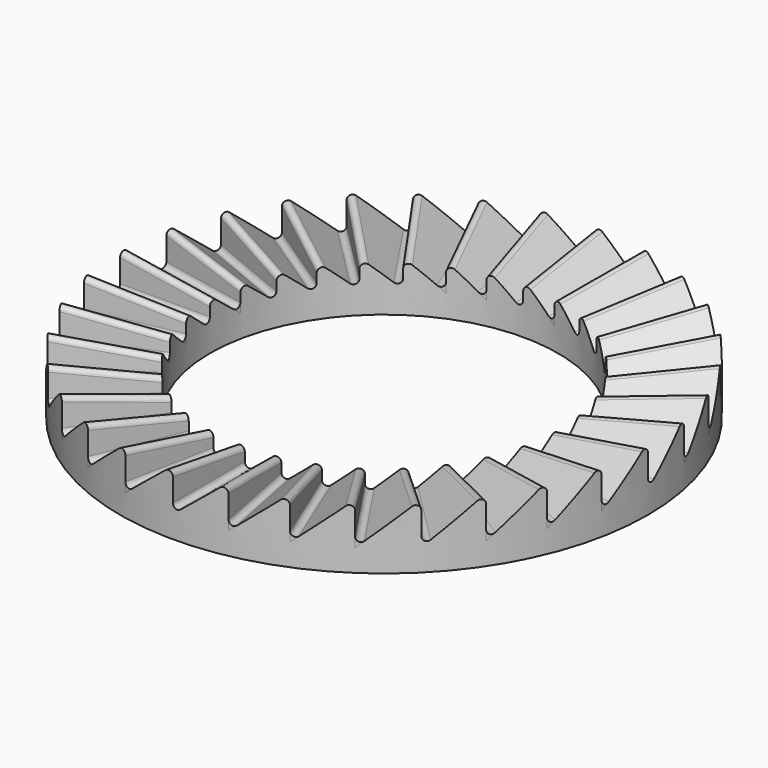
from build123d import *

# Parameters (mm, degrees)
F0_R          = 23.5
F0_R_2        = 15.5
F1_DEPTH      = 10
F3_DEPTH      = 23.5
F4_COUNT      = 32
F4_ANGLE      = 348.75
F7_T4_DEPTH   = 12.2119902172
F7_S5_R       = 23.5
F7_T6_DEPTH   = 8
F7_S7_R       = 15.5
F7_T8_DEPTH   = 8
F7_T12_DEPTH  = 12.2119902172
F7_S13_R      = 23.5
F7_T14_DEPTH  = 8
F7_S15_R      = 15.5
F7_T16_DEPTH  = 8
F7_T20_DEPTH  = 12.2119902172
F7_S21_R      = 23.5
F7_T22_DEPTH  = 8
F7_S23_R      = 15.5
F7_T24_DEPTH  = 8
F7_T28_DEPTH  = 12.2119902172
F7_S29_R      = 23.5
F7_T30_DEPTH  = 8
F7_S31_R      = 15.5
F7_T32_DEPTH  = 8
F7_T36_DEPTH  = 12.2119902172
F7_S37_R      = 23.5
F7_T38_DEPTH  = 8
F7_S39_R      = 15.5
F7_T40_DEPTH  = 8
F7_T44_DEPTH  = 12.2119902172
F7_S45_R      = 23.5
F7_T46_DEPTH  = 8
F7_S47_R      = 15.5
F7_T48_DEPTH  = 8
F7_T52_DEPTH  = 12.2119902172
F7_S53_R      = 23.5
F7_T54_DEPTH  = 8
F7_S55_R      = 15.5
F7_T56_DEPTH  = 8
F7_T60_DEPTH  = 12.2119902172
F7_S61_R      = 23.5
F7_T62_DEPTH  = 8
F7_S63_R      = 15.5
F7_T64_DEPTH  = 8
F7_T68_DEPTH  = 12.2119902172
F7_S69_R      = 23.5
F7_T70_DEPTH  = 8
F7_S71_R      = 15.5
F7_T72_DEPTH  = 8
F7_T76_DEPTH  = 12.2119902172
F7_S77_R      = 23.5
F7_T78_DEPTH  = 8
F7_S79_R      = 15.5
F7_T80_DEPTH  = 8
F7_T84_DEPTH  = 12.2119902172
F7_S85_R      = 23.5
F7_T86_DEPTH  = 8
F7_S87_R      = 15.5
F7_T88_DEPTH  = 8
F7_T92_DEPTH  = 12.2119902172
F7_S93_R      = 23.5
F7_T94_DEPTH  = 8
F7_S95_R      = 15.5
F7_T96_DEPTH  = 8
F7_T100_DEPTH = 12.2119902172
F7_S101_R     = 23.5
F7_T102_DEPTH = 8
F7_S103_R     = 15.5
F7_T104_DEPTH = 8
F7_T108_DEPTH = 12.2119902172
F7_S109_R     = 23.5
F7_T110_DEPTH = 8
F7_S111_R     = 15.5
F7_T112_DEPTH = 8
F7_T116_DEPTH = 12.2119902172
F7_S117_R     = 23.5
F7_T118_DEPTH = 8
F7_S119_R     = 15.5
F7_T120_DEPTH = 8
F7_T124_DEPTH = 12.2119902172
F7_S125_R     = 23.5
F7_T126_DEPTH = 8
F7_S127_R     = 15.5
F7_T128_DEPTH = 8
F7_T132_DEPTH = 12.2119902172
F7_S133_R     = 23.5
F7_T134_DEPTH = 8
F7_S135_R     = 15.5
F7_T136_DEPTH = 8
F7_T140_DEPTH = 12.2119902172
F7_S141_R     = 23.5
F7_T142_DEPTH = 8
F7_S143_R     = 15.5
F7_T144_DEPTH = 8
F7_T148_DEPTH = 12.2119902172
F7_S149_R     = 23.5
F7_T150_DEPTH = 8
F7_S151_R     = 15.5
F7_T152_DEPTH = 8
F7_T156_DEPTH = 12.2119902172
F7_S157_R     = 23.5
F7_T158_DEPTH = 8
F7_S159_R     = 15.5
F7_T160_DEPTH = 8
F7_T164_DEPTH = 12.2119902172
F7_S165_R     = 23.5
F7_T166_DEPTH = 8
F7_S167_R     = 15.5
F7_T168_DEPTH = 8
F7_T172_DEPTH = 12.2119902172
F7_S173_R     = 23.5
F7_T174_DEPTH = 8
F7_S175_R     = 15.5
F7_T176_DEPTH = 8
F7_T180_DEPTH = 12.2119902172
F7_S181_R     = 23.5
F7_T182_DEPTH = 8
F7_S183_R     = 15.5
F7_T184_DEPTH = 8
F7_T188_DEPTH = 12.2119902172
F7_S189_R     = 23.5
F7_T190_DEPTH = 8
F7_S191_R     = 15.5
F7_T192_DEPTH = 8
F7_T196_DEPTH = 12.2119902172
F7_S197_R     = 23.5
F7_T198_DEPTH = 8
F7_S199_R     = 15.5
F7_T200_DEPTH = 8
F7_T204_DEPTH = 12.2119902172
F7_S205_R     = 23.5
F7_T206_DEPTH = 8
F7_S207_R     = 15.5
F7_T208_DEPTH = 8
F7_T212_DEPTH = 12.2119902172
F7_S213_R     = 23.5
F7_T214_DEPTH = 8
F7_S215_R     = 15.5
F7_T216_DEPTH = 8
F7_T220_DEPTH = 12.2119902172
F7_S221_R     = 23.5
F7_T222_DEPTH = 8
F7_S223_R     = 15.5
F7_T224_DEPTH = 8
F7_T228_DEPTH = 12.2119902172
F7_S229_R     = 23.5
F7_T230_DEPTH = 8
F7_S231_R     = 15.5
F7_T232_DEPTH = 8
F7_T236_DEPTH = 12.2119902172
F7_S237_R     = 23.5
F7_T238_DEPTH = 8
F7_S239_R     = 15.5
F7_T240_DEPTH = 8
F7_T244_DEPTH = 12.2119902172
F7_S245_R     = 23.5
F7_T246_DEPTH = 8
F7_S247_R     = 15.5
F7_T248_DEPTH = 8
F7_T252_DEPTH = 12.2119902172
F7_S253_R     = 23.5
F7_T254_DEPTH = 8
F7_S255_R     = 15.5
F7_T256_DEPTH = 8
F7_T257_DEPTH = 12.2293454889
F7_T259_DEPTH = 12.2293454889
F7_T261_DEPTH = 12.2293454889
F7_T263_DEPTH = 12.2293454889
F7_T265_DEPTH = 12.2293454889
F7_T267_DEPTH = 12.2293454889
F7_T269_DEPTH = 12.2293454889
F7_T271_DEPTH = 12.2293454889
F7_T273_DEPTH = 12.2293454889
F7_T275_DEPTH = 12.2293454889
F7_T277_DEPTH = 12.2293454889
F7_T279_DEPTH = 12.2293454889
F7_T281_DEPTH = 12.2293454889
F7_T283_DEPTH = 12.2293454889
F7_T285_DEPTH = 12.2293454889
F7_T287_DEPTH = 12.2293454889
F7_T289_DEPTH = 12.2293454889
F7_T291_DEPTH = 12.2293454889
F7_T293_DEPTH = 12.2293454889
F7_T295_DEPTH = 12.2293454889
F7_T297_DEPTH = 12.2293454889
F7_T299_DEPTH = 12.2293454889
F7_T301_DEPTH = 12.2293454889
F7_T303_DEPTH = 12.2293454889
F7_T305_DEPTH = 12.2293454889
F7_T307_DEPTH = 12.2293454889
F7_T309_DEPTH = 12.2293454889
F7_T311_DEPTH = 12.2293454889
F7_T313_DEPTH = 12.2293454889
F7_T315_DEPTH = 12.2293454889
F7_T317_DEPTH = 12.2293454889
F7_T319_DEPTH = 12.2293454889


# Not quite as in the source:
# - a fillet or chamfer that OpenCascade refuses, or shapes differently, is made with other operations: its cross-section is extruded or revolved along the edge and cut away or added


with BuildPart() as f1:
    # F0 (on Top) → F1 (new body)
    with BuildSketch(Plane.XY):
        Circle(F0_R)
        Circle(F0_R_2, mode=Mode.SUBTRACT)
    extrude(amount=F1_DEPTH)


with BuildPart() as f3:
    # F2 (on Right) → F3 (new body)
    with BuildSketch(Plane.YZ):
        Polygon((9.808969115, 10.0010584846), (0, 10.0010584846), (0, 2.0010584846), align=None)
    extrude(amount=F3_DEPTH)


with BuildPart() as f4_1:
    # F4: instance of F3
    add(f3.part.rotate(Axis((0, 0, 6.0010584846), (0, 0, -1)), 1 * F4_ANGLE / (F4_COUNT - 1)))


with BuildPart() as f4_2:
    # F4: instance of F3
    add(f3.part.rotate(Axis((0, 0, 6.0010584846), (0, 0, -1)), 2 * F4_ANGLE / (F4_COUNT - 1)))


with BuildPart() as f4_3:
    # F4: instance of F3
    add(f3.part.rotate(Axis((0, 0, 6.0010584846), (0, 0, -1)), 3 * F4_ANGLE / (F4_COUNT - 1)))


with BuildPart() as f4_4:
    # F4: instance of F3
    add(f3.part.rotate(Axis((0, 0, 6.0010584846), (0, 0, -1)), 4 * F4_ANGLE / (F4_COUNT - 1)))


with BuildPart() as f4_5:
    # F4: instance of F3
    add(f3.part.rotate(Axis((0, 0, 6.0010584846), (0, 0, -1)), 5 * F4_ANGLE / (F4_COUNT - 1)))


with BuildPart() as f4_6:
    # F4: instance of F3
    add(f3.part.rotate(Axis((0, 0, 6.0010584846), (0, 0, -1)), 6 * F4_ANGLE / (F4_COUNT - 1)))


with BuildPart() as f4_7:
    # F4: instance of F3
    add(f3.part.rotate(Axis((0, 0, 6.0010584846), (0, 0, -1)), 7 * F4_ANGLE / (F4_COUNT - 1)))


with BuildPart() as f4_8:
    # F4: instance of F3
    add(f3.part.rotate(Axis((0, 0, 6.0010584846), (0, 0, -1)), 8 * F4_ANGLE / (F4_COUNT - 1)))


with BuildPart() as f4_9:
    # F4: instance of F3
    add(f3.part.rotate(Axis((0, 0, 6.0010584846), (0, 0, -1)), 9 * F4_ANGLE / (F4_COUNT - 1)))


with BuildPart() as f4_10:
    # F4: instance of F3
    add(f3.part.rotate(Axis((0, 0, 6.0010584846), (0, 0, -1)), 10 * F4_ANGLE / (F4_COUNT - 1)))


with BuildPart() as f4_11:
    # F4: instance of F3
    add(f3.part.rotate(Axis((0, 0, 6.0010584846), (0, 0, -1)), 11 * F4_ANGLE / (F4_COUNT - 1)))


with BuildPart() as f4_12:
    # F4: instance of F3
    add(f3.part.rotate(Axis((0, 0, 6.0010584846), (0, 0, -1)), 12 * F4_ANGLE / (F4_COUNT - 1)))


with BuildPart() as f4_13:
    # F4: instance of F3
    add(f3.part.rotate(Axis((0, 0, 6.0010584846), (0, 0, -1)), 13 * F4_ANGLE / (F4_COUNT - 1)))


with BuildPart() as f4_14:
    # F4: instance of F3
    add(f3.part.rotate(Axis((0, 0, 6.0010584846), (0, 0, -1)), 14 * F4_ANGLE / (F4_COUNT - 1)))


with BuildPart() as f4_15:
    # F4: instance of F3
    add(f3.part.rotate(Axis((0, 0, 6.0010584846), (0, 0, -1)), 15 * F4_ANGLE / (F4_COUNT - 1)))


with BuildPart() as f4_16:
    # F4: instance of F3
    add(f3.part.rotate(Axis((0, 0, 6.0010584846), (0, 0, -1)), 16 * F4_ANGLE / (F4_COUNT - 1)))


with BuildPart() as f4_17:
    # F4: instance of F3
    add(f3.part.rotate(Axis((0, 0, 6.0010584846), (0, 0, -1)), 17 * F4_ANGLE / (F4_COUNT - 1)))


with BuildPart() as f4_18:
    # F4: instance of F3
    add(f3.part.rotate(Axis((0, 0, 6.0010584846), (0, 0, -1)), 18 * F4_ANGLE / (F4_COUNT - 1)))


with BuildPart() as f4_19:
    # F4: instance of F3
    add(f3.part.rotate(Axis((0, 0, 6.0010584846), (0, 0, -1)), 19 * F4_ANGLE / (F4_COUNT - 1)))


with BuildPart() as f4_20:
    # F4: instance of F3
    add(f3.part.rotate(Axis((0, 0, 6.0010584846), (0, 0, -1)), 20 * F4_ANGLE / (F4_COUNT - 1)))


with BuildPart() as f4_21:
    # F4: instance of F3
    add(f3.part.rotate(Axis((0, 0, 6.0010584846), (0, 0, -1)), 21 * F4_ANGLE / (F4_COUNT - 1)))


with BuildPart() as f4_22:
    # F4: instance of F3
    add(f3.part.rotate(Axis((0, 0, 6.0010584846), (0, 0, -1)), 22 * F4_ANGLE / (F4_COUNT - 1)))


with BuildPart() as f4_23:
    # F4: instance of F3
    add(f3.part.rotate(Axis((0, 0, 6.0010584846), (0, 0, -1)), 23 * F4_ANGLE / (F4_COUNT - 1)))


with BuildPart() as f4_24:
    # F4: instance of F3
    add(f3.part.rotate(Axis((0, 0, 6.0010584846), (0, 0, -1)), 24 * F4_ANGLE / (F4_COUNT - 1)))


with BuildPart() as f4_25:
    # F4: instance of F3
    add(f3.part.rotate(Axis((0, 0, 6.0010584846), (0, 0, -1)), 25 * F4_ANGLE / (F4_COUNT - 1)))


with BuildPart() as f4_26:
    # F4: instance of F3
    add(f3.part.rotate(Axis((0, 0, 6.0010584846), (0, 0, -1)), 26 * F4_ANGLE / (F4_COUNT - 1)))


with BuildPart() as f4_27:
    # F4: instance of F3
    add(f3.part.rotate(Axis((0, 0, 6.0010584846), (0, 0, -1)), 27 * F4_ANGLE / (F4_COUNT - 1)))


with BuildPart() as f4_28:
    # F4: instance of F3
    add(f3.part.rotate(Axis((0, 0, 6.0010584846), (0, 0, -1)), 28 * F4_ANGLE / (F4_COUNT - 1)))


with BuildPart() as f4_29:
    # F4: instance of F3
    add(f3.part.rotate(Axis((0, 0, 6.0010584846), (0, 0, -1)), 29 * F4_ANGLE / (F4_COUNT - 1)))


with BuildPart() as f4_30:
    # F4: instance of F3
    add(f3.part.rotate(Axis((0, 0, 6.0010584846), (0, 0, -1)), 30 * F4_ANGLE / (F4_COUNT - 1)))


with BuildPart() as f4_31:
    # F4: instance of F3
    add(f3.part.rotate(Axis((0, 0, 6.0010584846), (0, 0, -1)), 31 * F4_ANGLE / (F4_COUNT - 1)))


with BuildPart() as f3_1:
    add(f3.part)

    # F5: union F4_1, F4_2, F4_3, F4_4, F4_5, F4_6, F4_7, F4_8, F4_9, F4_10, F4_11, F4_12, F4_13, F4_14, F4_15, F4_16, F4_17, F4_18, F4_19, F4_20, F4_21, F4_22, F4_23, F4_24, F4_25, F4_26, F4_27, F4_28, F4_29, F4_30, F4_31
    add(f4_1.part)
    add(f4_2.part)
    add(f4_3.part)
    add(f4_4.part)
    add(f4_5.part)
    add(f4_6.part)
    add(f4_7.part)
    add(f4_8.part)
    add(f4_9.part)
    add(f4_10.part)
    add(f4_11.part)
    add(f4_12.part)
    add(f4_13.part)
    add(f4_14.part)
    add(f4_15.part)
    add(f4_16.part)
    add(f4_17.part)
    add(f4_18.part)
    add(f4_19.part)
    add(f4_20.part)
    add(f4_21.part)
    add(f4_22.part)
    add(f4_23.part)
    add(f4_24.part)
    add(f4_25.part)
    add(f4_26.part)
    add(f4_27.part)
    add(f4_28.part)
    add(f4_29.part)
    add(f4_30.part)
    add(f4_31.part)


with BuildPart() as f1_1:
    add(f1.part)

    # F6: cut F3
    add(f3_1.part, mode=Mode.SUBTRACT)

    # F7: fillet of radius 0.4 on 64 edges, made by hand


with BuildPart() as f7_tool2:
    # F7_s3 → F7_t4 (new body)
    with BuildSketch(Plane(origin=(5.1256637649, -12.3744469775, 0), x_dir=(0, 0, 1), z_dir=(0.3826834324, -0.9238795325, 0))):
        with BuildLine():
            add(Edge.make_bspline(
                [(2.5334787325, -0.6528117211), (2.0010584846, 0), (2.843456528, 0)],
                knots=[0, 0, 0, 1, 1, 1], degree=2, weights=[1, 0.4285714286, 1]))
            Line((2.843456528, 0), (2.0010584846, 0))
            Line((2.0010584846, 0), (2.5334787325, -0.6528117211))
        make_face()
    extrude(amount=F7_T4_DEPTH)

    # F7_s5 → F7_t6 (intersect, symmetric)
    with BuildSketch(Plane.XY.offset(2.4)):
        Circle(F7_S5_R)
    extrude(amount=F7_T6_DEPTH, both=True, mode=Mode.INTERSECT)

    # F7_s7 → F7_t8 (cut, symmetric)
    with BuildSketch(Plane.XY.offset(2.4)):
        Circle(F7_S7_R)
    extrude(amount=F7_T8_DEPTH, both=True, mode=Mode.SUBTRACT)


with BuildPart() as f1_2:
    add(f1_1.part)

    # F7_t1: union F7_tool2
    add(f7_tool2.part)


with BuildPart() as f7_tool10:
    # F7_s11 → F7_t12 (new body)
    with BuildSketch(Plane(origin=(7.4413104186, -11.1367080542, 0), x_dir=(0, 0, 1), z_dir=(0.555570233, -0.8314696123, 0))):
        with BuildLine():
            add(Edge.make_bspline(
                [(2.5334787325, -0.6528117211), (2.0010584846, 0), (2.843456528, 0)],
                knots=[0, 0, 0, 1, 1, 1], degree=2, weights=[1, 0.4285714286, 1]))
            Line((2.843456528, 0), (2.0010584846, 0))
            Line((2.0010584846, 0), (2.5334787325, -0.6528117211))
        make_face()
    extrude(amount=F7_T12_DEPTH)

    # F7_s13 → F7_t14 (intersect, symmetric)
    with BuildSketch(Plane.XY.offset(2.4)):
        Circle(F7_S13_R)
    extrude(amount=F7_T14_DEPTH, both=True, mode=Mode.INTERSECT)

    # F7_s15 → F7_t16 (cut, symmetric)
    with BuildSketch(Plane.XY.offset(2.4)):
        Circle(F7_S15_R)
    extrude(amount=F7_T16_DEPTH, both=True, mode=Mode.SUBTRACT)


with BuildPart() as f1_3:
    add(f1_2.part)

    # F7_t9: union F7_tool10
    add(f7_tool10.part)


with BuildPart() as f7_tool18:
    # F7_s19 → F7_t20 (new body)
    with BuildSketch(Plane(origin=(9.4709916859, -9.4709916859, 0), x_dir=(0, 0, 1), z_dir=(0.7071067812, -0.7071067812, 0))):
        with BuildLine():
            add(Edge.make_bspline(
                [(2.5334787325, -0.6528117211), (2.0010584846, 0), (2.843456528, 0)],
                knots=[0, 0, 0, 1, 1, 1], degree=2, weights=[1, 0.4285714286, 1]))
            Line((2.843456528, 0), (2.0010584846, 0))
            Line((2.0010584846, 0), (2.5334787325, -0.6528117211))
        make_face()
    extrude(amount=F7_T20_DEPTH)

    # F7_s21 → F7_t22 (intersect, symmetric)
    with BuildSketch(Plane.XY.offset(2.4)):
        Circle(F7_S21_R)
    extrude(amount=F7_T22_DEPTH, both=True, mode=Mode.INTERSECT)

    # F7_s23 → F7_t24 (cut, symmetric)
    with BuildSketch(Plane.XY.offset(2.4)):
        Circle(F7_S23_R)
    extrude(amount=F7_T24_DEPTH, both=True, mode=Mode.SUBTRACT)


with BuildPart() as f1_4:
    add(f1_3.part)

    # F7_t17: union F7_tool18
    add(f7_tool18.part)


with BuildPart() as f7_tool26:
    # F7_s27 → F7_t28 (new body)
    with BuildSketch(Plane(origin=(11.1367080542, -7.4413104186, 0), x_dir=(0, 0, 1), z_dir=(0.8314696123, -0.555570233, 0))):
        with BuildLine():
            add(Edge.make_bspline(
                [(2.5334787325, -0.6528117211), (2.0010584846, 0), (2.843456528, 0)],
                knots=[0, 0, 0, 1, 1, 1], degree=2, weights=[1, 0.4285714286, 1]))
            Line((2.843456528, 0), (2.0010584846, 0))
            Line((2.0010584846, 0), (2.5334787325, -0.6528117211))
        make_face()
    extrude(amount=F7_T28_DEPTH)

    # F7_s29 → F7_t30 (intersect, symmetric)
    with BuildSketch(Plane.XY.offset(2.4)):
        Circle(F7_S29_R)
    extrude(amount=F7_T30_DEPTH, both=True, mode=Mode.INTERSECT)

    # F7_s31 → F7_t32 (cut, symmetric)
    with BuildSketch(Plane.XY.offset(2.4)):
        Circle(F7_S31_R)
    extrude(amount=F7_T32_DEPTH, both=True, mode=Mode.SUBTRACT)


with BuildPart() as f1_5:
    add(f1_4.part)

    # F7_t25: union F7_tool26
    add(f7_tool26.part)


with BuildPart() as f7_tool34:
    # F7_s35 → F7_t36 (new body)
    with BuildSketch(Plane(origin=(12.3744469775, -5.1256637649, 0), x_dir=(0, 0, 1), z_dir=(0.9238795325, -0.3826834324, 0))):
        with BuildLine():
            add(Edge.make_bspline(
                [(2.5334787325, -0.6528117211), (2.0010584846, 0), (2.843456528, 0)],
                knots=[0, 0, 0, 1, 1, 1], degree=2, weights=[1, 0.4285714286, 1]))
            Line((2.843456528, 0), (2.0010584846, 0))
            Line((2.0010584846, 0), (2.5334787325, -0.6528117211))
        make_face()
    extrude(amount=F7_T36_DEPTH)

    # F7_s37 → F7_t38 (intersect, symmetric)
    with BuildSketch(Plane.XY.offset(2.4)):
        Circle(F7_S37_R)
    extrude(amount=F7_T38_DEPTH, both=True, mode=Mode.INTERSECT)

    # F7_s39 → F7_t40 (cut, symmetric)
    with BuildSketch(Plane.XY.offset(2.4)):
        Circle(F7_S39_R)
    extrude(amount=F7_T40_DEPTH, both=True, mode=Mode.SUBTRACT)


with BuildPart() as f1_6:
    add(f1_5.part)

    # F7_t33: union F7_tool34
    add(f7_tool34.part)


with BuildPart() as f7_tool42:
    # F7_s43 → F7_t44 (new body)
    with BuildSketch(Plane(origin=(13.1366428431, -2.6130407273, 0), x_dir=(0, 0, 1), z_dir=(0.9807852804, -0.195090322, 0))):
        with BuildLine():
            add(Edge.make_bspline(
                [(2.5334787325, -0.6528117211), (2.0010584846, 0), (2.843456528, 0)],
                knots=[0, 0, 0, 1, 1, 1], degree=2, weights=[1, 0.4285714286, 1]))
            Line((2.843456528, 0), (2.0010584846, 0))
            Line((2.0010584846, 0), (2.5334787325, -0.6528117211))
        make_face()
    extrude(amount=F7_T44_DEPTH)

    # F7_s45 → F7_t46 (intersect, symmetric)
    with BuildSketch(Plane.XY.offset(2.4)):
        Circle(F7_S45_R)
    extrude(amount=F7_T46_DEPTH, both=True, mode=Mode.INTERSECT)

    # F7_s47 → F7_t48 (cut, symmetric)
    with BuildSketch(Plane.XY.offset(2.4)):
        Circle(F7_S47_R)
    extrude(amount=F7_T48_DEPTH, both=True, mode=Mode.SUBTRACT)


with BuildPart() as f1_7:
    add(f1_6.part)

    # F7_t41: union F7_tool42
    add(f7_tool42.part)


with BuildPart() as f7_tool50:
    # F7_s51 → F7_t52 (new body)
    with BuildSketch(Plane.YZ.offset(13.3940048914)):
        with BuildLine():
            add(Edge.make_bspline(
                [(0, 2.843456528), (0, 2.0010584846), (0.6528117211, 2.5334787325)],
                knots=[0, 0, 0, 1, 1, 1], degree=2, weights=[1, 0.4285714286, 1]))
            Line((0.6528117211, 2.5334787325), (0, 2.0010584846))
            Line((0, 2.0010584846), (0, 2.843456528))
        make_face()
    extrude(amount=F7_T52_DEPTH)

    # F7_s53 → F7_t54 (intersect, symmetric)
    with BuildSketch(Plane.XY.offset(2.4)):
        Circle(F7_S53_R)
    extrude(amount=F7_T54_DEPTH, both=True, mode=Mode.INTERSECT)

    # F7_s55 → F7_t56 (cut, symmetric)
    with BuildSketch(Plane.XY.offset(2.4)):
        Circle(F7_S55_R)
    extrude(amount=F7_T56_DEPTH, both=True, mode=Mode.SUBTRACT)


with BuildPart() as f1_8:
    add(f1_7.part)

    # F7_t49: union F7_tool50
    add(f7_tool50.part)


with BuildPart() as f7_tool58:
    # F7_s59 → F7_t60 (new body)
    with BuildSketch(Plane(origin=(13.1366428431, 2.6130407273, 0), x_dir=(0, 0, 1), z_dir=(0.9807852804, 0.195090322, 0))):
        with BuildLine():
            add(Edge.make_bspline(
                [(2.5334787325, -0.6528117211), (2.0010584846, 0), (2.843456528, 0)],
                knots=[0, 0, 0, 1, 1, 1], degree=2, weights=[1, 0.4285714286, 1]))
            Line((2.843456528, 0), (2.0010584846, 0))
            Line((2.0010584846, 0), (2.5334787325, -0.6528117211))
        make_face()
    extrude(amount=F7_T60_DEPTH)

    # F7_s61 → F7_t62 (intersect, symmetric)
    with BuildSketch(Plane.XY.offset(2.4)):
        Circle(F7_S61_R)
    extrude(amount=F7_T62_DEPTH, both=True, mode=Mode.INTERSECT)

    # F7_s63 → F7_t64 (cut, symmetric)
    with BuildSketch(Plane.XY.offset(2.4)):
        Circle(F7_S63_R)
    extrude(amount=F7_T64_DEPTH, both=True, mode=Mode.SUBTRACT)


with BuildPart() as f1_9:
    add(f1_8.part)

    # F7_t57: union F7_tool58
    add(f7_tool58.part)


with BuildPart() as f7_tool66:
    # F7_s67 → F7_t68 (new body)
    with BuildSketch(Plane(origin=(11.1367080542, 7.4413104186, 0), x_dir=(0, 0, 1), z_dir=(0.8314696123, 0.555570233, 0))):
        with BuildLine():
            add(Edge.make_bspline(
                [(2.5334787325, -0.6528117211), (2.0010584846, 0), (2.843456528, 0)],
                knots=[0, 0, 0, 1, 1, 1], degree=2, weights=[1, 0.4285714286, 1]))
            Line((2.843456528, 0), (2.0010584846, 0))
            Line((2.0010584846, 0), (2.5334787325, -0.6528117211))
        make_face()
    extrude(amount=F7_T68_DEPTH)

    # F7_s69 → F7_t70 (intersect, symmetric)
    with BuildSketch(Plane.XY.offset(2.4)):
        Circle(F7_S69_R)
    extrude(amount=F7_T70_DEPTH, both=True, mode=Mode.INTERSECT)

    # F7_s71 → F7_t72 (cut, symmetric)
    with BuildSketch(Plane.XY.offset(2.4)):
        Circle(F7_S71_R)
    extrude(amount=F7_T72_DEPTH, both=True, mode=Mode.SUBTRACT)


with BuildPart() as f1_10:
    add(f1_9.part)

    # F7_t65: union F7_tool66
    add(f7_tool66.part)


with BuildPart() as f7_tool74:
    # F7_s75 → F7_t76 (new body)
    with BuildSketch(Plane(origin=(12.3744469775, 5.1256637649, 0), x_dir=(0, 0, 1), z_dir=(0.9238795325, 0.3826834324, 0))):
        with BuildLine():
            add(Edge.make_bspline(
                [(2.5334787325, -0.6528117211), (2.0010584846, 0), (2.843456528, 0)],
                knots=[0, 0, 0, 1, 1, 1], degree=2, weights=[1, 0.4285714286, 1]))
            Line((2.843456528, 0), (2.0010584846, 0))
            Line((2.0010584846, 0), (2.5334787325, -0.6528117211))
        make_face()
    extrude(amount=F7_T76_DEPTH)

    # F7_s77 → F7_t78 (intersect, symmetric)
    with BuildSketch(Plane.XY.offset(2.4)):
        Circle(F7_S77_R)
    extrude(amount=F7_T78_DEPTH, both=True, mode=Mode.INTERSECT)

    # F7_s79 → F7_t80 (cut, symmetric)
    with BuildSketch(Plane.XY.offset(2.4)):
        Circle(F7_S79_R)
    extrude(amount=F7_T80_DEPTH, both=True, mode=Mode.SUBTRACT)


with BuildPart() as f1_11:
    add(f1_10.part)

    # F7_t73: union F7_tool74
    add(f7_tool74.part)


with BuildPart() as f7_tool82:
    # F7_s83 → F7_t84 (new body)
    with BuildSketch(Plane(origin=(9.4709916859, 9.4709916859, 0), x_dir=(0, 0, 1), z_dir=(0.7071067812, 0.7071067812, 0))):
        with BuildLine():
            add(Edge.make_bspline(
                [(2.5334787325, -0.6528117211), (2.0010584846, 0), (2.843456528, 0)],
                knots=[0, 0, 0, 1, 1, 1], degree=2, weights=[1, 0.4285714286, 1]))
            Line((2.843456528, 0), (2.0010584846, 0))
            Line((2.0010584846, 0), (2.5334787325, -0.6528117211))
        make_face()
    extrude(amount=F7_T84_DEPTH)

    # F7_s85 → F7_t86 (intersect, symmetric)
    with BuildSketch(Plane.XY.offset(2.4)):
        Circle(F7_S85_R)
    extrude(amount=F7_T86_DEPTH, both=True, mode=Mode.INTERSECT)

    # F7_s87 → F7_t88 (cut, symmetric)
    with BuildSketch(Plane.XY.offset(2.4)):
        Circle(F7_S87_R)
    extrude(amount=F7_T88_DEPTH, both=True, mode=Mode.SUBTRACT)


with BuildPart() as f1_12:
    add(f1_11.part)

    # F7_t81: union F7_tool82
    add(f7_tool82.part)


with BuildPart() as f7_tool90:
    # F7_s91 → F7_t92 (new body)
    with BuildSketch(Plane(origin=(7.4413104186, 11.1367080542, 0), x_dir=(0, 0, 1), z_dir=(0.555570233, 0.8314696123, 0))):
        with BuildLine():
            add(Edge.make_bspline(
                [(2.5334787325, -0.6528117211), (2.0010584846, 0), (2.843456528, 0)],
                knots=[0, 0, 0, 1, 1, 1], degree=2, weights=[1, 0.4285714286, 1]))
            Line((2.843456528, 0), (2.0010584846, 0))
            Line((2.0010584846, 0), (2.5334787325, -0.6528117211))
        make_face()
    extrude(amount=F7_T92_DEPTH)

    # F7_s93 → F7_t94 (intersect, symmetric)
    with BuildSketch(Plane.XY.offset(2.4)):
        Circle(F7_S93_R)
    extrude(amount=F7_T94_DEPTH, both=True, mode=Mode.INTERSECT)

    # F7_s95 → F7_t96 (cut, symmetric)
    with BuildSketch(Plane.XY.offset(2.4)):
        Circle(F7_S95_R)
    extrude(amount=F7_T96_DEPTH, both=True, mode=Mode.SUBTRACT)


with BuildPart() as f1_13:
    add(f1_12.part)

    # F7_t89: union F7_tool90
    add(f7_tool90.part)


with BuildPart() as f7_tool98:
    # F7_s99 → F7_t100 (new body)
    with BuildSketch(Plane(origin=(5.1256637649, 12.3744469775, 0), x_dir=(0, 0, 1), z_dir=(0.3826834324, 0.9238795325, 0))):
        with BuildLine():
            add(Edge.make_bspline(
                [(2.5334787325, -0.6528117211), (2.0010584846, 0), (2.843456528, 0)],
                knots=[0, 0, 0, 1, 1, 1], degree=2, weights=[1, 0.4285714286, 1]))
            Line((2.843456528, 0), (2.0010584846, 0))
            Line((2.0010584846, 0), (2.5334787325, -0.6528117211))
        make_face()
    extrude(amount=F7_T100_DEPTH)

    # F7_s101 → F7_t102 (intersect, symmetric)
    with BuildSketch(Plane.XY.offset(2.4)):
        Circle(F7_S101_R)
    extrude(amount=F7_T102_DEPTH, both=True, mode=Mode.INTERSECT)

    # F7_s103 → F7_t104 (cut, symmetric)
    with BuildSketch(Plane.XY.offset(2.4)):
        Circle(F7_S103_R)
    extrude(amount=F7_T104_DEPTH, both=True, mode=Mode.SUBTRACT)


with BuildPart() as f1_14:
    add(f1_13.part)

    # F7_t97: union F7_tool98
    add(f7_tool98.part)


with BuildPart() as f7_tool106:
    # F7_s107 → F7_t108 (new body)
    with BuildSketch(Plane(origin=(2.6130407273, 13.1366428431, 0), x_dir=(0, 0, 1), z_dir=(0.195090322, 0.9807852804, 0))):
        with BuildLine():
            add(Edge.make_bspline(
                [(2.5334787325, -0.6528117211), (2.0010584846, 0), (2.843456528, 0)],
                knots=[0, 0, 0, 1, 1, 1], degree=2, weights=[1, 0.4285714286, 1]))
            Line((2.843456528, 0), (2.0010584846, 0))
            Line((2.0010584846, 0), (2.5334787325, -0.6528117211))
        make_face()
    extrude(amount=F7_T108_DEPTH)

    # F7_s109 → F7_t110 (intersect, symmetric)
    with BuildSketch(Plane.XY.offset(2.4)):
        Circle(F7_S109_R)
    extrude(amount=F7_T110_DEPTH, both=True, mode=Mode.INTERSECT)

    # F7_s111 → F7_t112 (cut, symmetric)
    with BuildSketch(Plane.XY.offset(2.4)):
        Circle(F7_S111_R)
    extrude(amount=F7_T112_DEPTH, both=True, mode=Mode.SUBTRACT)


with BuildPart() as f1_15:
    add(f1_14.part)

    # F7_t105: union F7_tool106
    add(f7_tool106.part)


with BuildPart() as f7_tool114:
    # F7_s115 → F7_t116 (new body)
    with BuildSketch(Plane.XZ.offset(-13.3940048914)):
        with BuildLine():
            add(Edge.make_bspline(
                [(-0.6528117211, 2.5334787325), (0, 2.0010584846), (0, 2.843456528)],
                knots=[0, 0, 0, 1, 1, 1], degree=2, weights=[1, 0.4285714286, 1]))
            Line((0, 2.843456528), (0, 2.0010584846))
            Line((0, 2.0010584846), (-0.6528117211, 2.5334787325))
        make_face()
    extrude(amount=-F7_T116_DEPTH)

    # F7_s117 → F7_t118 (intersect, symmetric)
    with BuildSketch(Plane.XY.offset(2.4)):
        Circle(F7_S117_R)
    extrude(amount=F7_T118_DEPTH, both=True, mode=Mode.INTERSECT)

    # F7_s119 → F7_t120 (cut, symmetric)
    with BuildSketch(Plane.XY.offset(2.4)):
        Circle(F7_S119_R)
    extrude(amount=F7_T120_DEPTH, both=True, mode=Mode.SUBTRACT)


with BuildPart() as f1_16:
    add(f1_15.part)

    # F7_t113: union F7_tool114
    add(f7_tool114.part)


with BuildPart() as f7_tool122:
    # F7_s123 → F7_t124 (new body)
    with BuildSketch(Plane(origin=(-2.6130407273, 13.1366428431, 0), x_dir=(0, 0, 1), z_dir=(-0.195090322, 0.9807852804, 0))):
        with BuildLine():
            add(Edge.make_bspline(
                [(2.5334787325, -0.6528117211), (2.0010584846, 0), (2.843456528, 0)],
                knots=[0, 0, 0, 1, 1, 1], degree=2, weights=[1, 0.4285714286, 1]))
            Line((2.843456528, 0), (2.0010584846, 0))
            Line((2.0010584846, 0), (2.5334787325, -0.6528117211))
        make_face()
    extrude(amount=F7_T124_DEPTH)

    # F7_s125 → F7_t126 (intersect, symmetric)
    with BuildSketch(Plane.XY.offset(2.4)):
        Circle(F7_S125_R)
    extrude(amount=F7_T126_DEPTH, both=True, mode=Mode.INTERSECT)

    # F7_s127 → F7_t128 (cut, symmetric)
    with BuildSketch(Plane.XY.offset(2.4)):
        Circle(F7_S127_R)
    extrude(amount=F7_T128_DEPTH, both=True, mode=Mode.SUBTRACT)


with BuildPart() as f1_17:
    add(f1_16.part)

    # F7_t121: union F7_tool122
    add(f7_tool122.part)


with BuildPart() as f7_tool130:
    # F7_s131 → F7_t132 (new body)
    with BuildSketch(Plane(origin=(-5.1256637649, 12.3744469775, 0), x_dir=(0, 0, 1), z_dir=(-0.3826834324, 0.9238795325, 0))):
        with BuildLine():
            add(Edge.make_bspline(
                [(2.5334787325, -0.6528117211), (2.0010584846, 0), (2.843456528, 0)],
                knots=[0, 0, 0, 1, 1, 1], degree=2, weights=[1, 0.4285714286, 1]))
            Line((2.843456528, 0), (2.0010584846, 0))
            Line((2.0010584846, 0), (2.5334787325, -0.6528117211))
        make_face()
    extrude(amount=F7_T132_DEPTH)

    # F7_s133 → F7_t134 (intersect, symmetric)
    with BuildSketch(Plane.XY.offset(2.4)):
        Circle(F7_S133_R)
    extrude(amount=F7_T134_DEPTH, both=True, mode=Mode.INTERSECT)

    # F7_s135 → F7_t136 (cut, symmetric)
    with BuildSketch(Plane.XY.offset(2.4)):
        Circle(F7_S135_R)
    extrude(amount=F7_T136_DEPTH, both=True, mode=Mode.SUBTRACT)


with BuildPart() as f1_18:
    add(f1_17.part)

    # F7_t129: union F7_tool130
    add(f7_tool130.part)


with BuildPart() as f7_tool138:
    # F7_s139 → F7_t140 (new body)
    with BuildSketch(Plane(origin=(-7.4413104186, 11.1367080542, 0), x_dir=(0, 0, 1), z_dir=(-0.555570233, 0.8314696123, 0))):
        with BuildLine():
            add(Edge.make_bspline(
                [(2.5334787325, -0.6528117211), (2.0010584846, 0), (2.843456528, 0)],
                knots=[0, 0, 0, 1, 1, 1], degree=2, weights=[1, 0.4285714286, 1]))
            Line((2.843456528, 0), (2.0010584846, 0))
            Line((2.0010584846, 0), (2.5334787325, -0.6528117211))
        make_face()
    extrude(amount=F7_T140_DEPTH)

    # F7_s141 → F7_t142 (intersect, symmetric)
    with BuildSketch(Plane.XY.offset(2.4)):
        Circle(F7_S141_R)
    extrude(amount=F7_T142_DEPTH, both=True, mode=Mode.INTERSECT)

    # F7_s143 → F7_t144 (cut, symmetric)
    with BuildSketch(Plane.XY.offset(2.4)):
        Circle(F7_S143_R)
    extrude(amount=F7_T144_DEPTH, both=True, mode=Mode.SUBTRACT)


with BuildPart() as f1_19:
    add(f1_18.part)

    # F7_t137: union F7_tool138
    add(f7_tool138.part)


with BuildPart() as f7_tool146:
    # F7_s147 → F7_t148 (new body)
    with BuildSketch(Plane(origin=(-9.4709916859, 9.4709916859, 0), x_dir=(0, 0, 1), z_dir=(-0.7071067812, 0.7071067812, 0))):
        with BuildLine():
            add(Edge.make_bspline(
                [(2.5334787325, -0.6528117211), (2.0010584846, 0), (2.843456528, 0)],
                knots=[0, 0, 0, 1, 1, 1], degree=2, weights=[1, 0.4285714286, 1]))
            Line((2.843456528, 0), (2.0010584846, 0))
            Line((2.0010584846, 0), (2.5334787325, -0.6528117211))
        make_face()
    extrude(amount=F7_T148_DEPTH)

    # F7_s149 → F7_t150 (intersect, symmetric)
    with BuildSketch(Plane.XY.offset(2.4)):
        Circle(F7_S149_R)
    extrude(amount=F7_T150_DEPTH, both=True, mode=Mode.INTERSECT)

    # F7_s151 → F7_t152 (cut, symmetric)
    with BuildSketch(Plane.XY.offset(2.4)):
        Circle(F7_S151_R)
    extrude(amount=F7_T152_DEPTH, both=True, mode=Mode.SUBTRACT)


with BuildPart() as f1_20:
    add(f1_19.part)

    # F7_t145: union F7_tool146
    add(f7_tool146.part)


with BuildPart() as f7_tool154:
    # F7_s155 → F7_t156 (new body)
    with BuildSketch(Plane(origin=(-11.1367080542, 7.4413104186, 0), x_dir=(0, 0, 1), z_dir=(-0.8314696123, 0.555570233, 0))):
        with BuildLine():
            add(Edge.make_bspline(
                [(2.5334787325, -0.6528117211), (2.0010584846, 0), (2.843456528, 0)],
                knots=[0, 0, 0, 1, 1, 1], degree=2, weights=[1, 0.4285714286, 1]))
            Line((2.843456528, 0), (2.0010584846, 0))
            Line((2.0010584846, 0), (2.5334787325, -0.6528117211))
        make_face()
    extrude(amount=F7_T156_DEPTH)

    # F7_s157 → F7_t158 (intersect, symmetric)
    with BuildSketch(Plane.XY.offset(2.4)):
        Circle(F7_S157_R)
    extrude(amount=F7_T158_DEPTH, both=True, mode=Mode.INTERSECT)

    # F7_s159 → F7_t160 (cut, symmetric)
    with BuildSketch(Plane.XY.offset(2.4)):
        Circle(F7_S159_R)
    extrude(amount=F7_T160_DEPTH, both=True, mode=Mode.SUBTRACT)


with BuildPart() as f1_21:
    add(f1_20.part)

    # F7_t153: union F7_tool154
    add(f7_tool154.part)


with BuildPart() as f7_tool162:
    # F7_s163 → F7_t164 (new body)
    with BuildSketch(Plane(origin=(-12.3744469775, 5.1256637649, 0), x_dir=(0, 0, 1), z_dir=(-0.9238795325, 0.3826834324, 0))):
        with BuildLine():
            add(Edge.make_bspline(
                [(2.5334787325, -0.6528117211), (2.0010584846, 0), (2.843456528, 0)],
                knots=[0, 0, 0, 1, 1, 1], degree=2, weights=[1, 0.4285714286, 1]))
            Line((2.843456528, 0), (2.0010584846, 0))
            Line((2.0010584846, 0), (2.5334787325, -0.6528117211))
        make_face()
    extrude(amount=F7_T164_DEPTH)

    # F7_s165 → F7_t166 (intersect, symmetric)
    with BuildSketch(Plane.XY.offset(2.4)):
        Circle(F7_S165_R)
    extrude(amount=F7_T166_DEPTH, both=True, mode=Mode.INTERSECT)

    # F7_s167 → F7_t168 (cut, symmetric)
    with BuildSketch(Plane.XY.offset(2.4)):
        Circle(F7_S167_R)
    extrude(amount=F7_T168_DEPTH, both=True, mode=Mode.SUBTRACT)


with BuildPart() as f1_22:
    add(f1_21.part)

    # F7_t161: union F7_tool162
    add(f7_tool162.part)


with BuildPart() as f7_tool170:
    # F7_s171 → F7_t172 (new body)
    with BuildSketch(Plane(origin=(-13.1366428431, 2.6130407273, 0), x_dir=(0, 0, 1), z_dir=(-0.9807852804, 0.195090322, 0))):
        with BuildLine():
            add(Edge.make_bspline(
                [(2.5334787325, -0.6528117211), (2.0010584846, 0), (2.843456528, 0)],
                knots=[0, 0, 0, 1, 1, 1], degree=2, weights=[1, 0.4285714286, 1]))
            Line((2.843456528, 0), (2.0010584846, 0))
            Line((2.0010584846, 0), (2.5334787325, -0.6528117211))
        make_face()
    extrude(amount=F7_T172_DEPTH)

    # F7_s173 → F7_t174 (intersect, symmetric)
    with BuildSketch(Plane.XY.offset(2.4)):
        Circle(F7_S173_R)
    extrude(amount=F7_T174_DEPTH, both=True, mode=Mode.INTERSECT)

    # F7_s175 → F7_t176 (cut, symmetric)
    with BuildSketch(Plane.XY.offset(2.4)):
        Circle(F7_S175_R)
    extrude(amount=F7_T176_DEPTH, both=True, mode=Mode.SUBTRACT)


with BuildPart() as f1_23:
    add(f1_22.part)

    # F7_t169: union F7_tool170
    add(f7_tool170.part)


with BuildPart() as f7_tool178:
    # F7_s179 → F7_t180 (new body)
    with BuildSketch(Plane.YZ.offset(-13.3940048914)):
        with BuildLine():
            add(Edge.make_bspline(
                [(-0.6528117211, 2.5334787325), (0, 2.0010584846), (0, 2.843456528)],
                knots=[0, 0, 0, 1, 1, 1], degree=2, weights=[1, 0.4285714286, 1]))
            Line((0, 2.843456528), (0, 2.0010584846))
            Line((0, 2.0010584846), (-0.6528117211, 2.5334787325))
        make_face()
    extrude(amount=-F7_T180_DEPTH)

    # F7_s181 → F7_t182 (intersect, symmetric)
    with BuildSketch(Plane.XY.offset(2.4)):
        Circle(F7_S181_R)
    extrude(amount=F7_T182_DEPTH, both=True, mode=Mode.INTERSECT)

    # F7_s183 → F7_t184 (cut, symmetric)
    with BuildSketch(Plane.XY.offset(2.4)):
        Circle(F7_S183_R)
    extrude(amount=F7_T184_DEPTH, both=True, mode=Mode.SUBTRACT)


with BuildPart() as f1_24:
    add(f1_23.part)

    # F7_t177: union F7_tool178
    add(f7_tool178.part)


with BuildPart() as f7_tool186:
    # F7_s187 → F7_t188 (new body)
    with BuildSketch(Plane(origin=(-13.1366428431, -2.6130407273, 0), x_dir=(0, 0, 1), z_dir=(-0.9807852804, -0.195090322, 0))):
        with BuildLine():
            add(Edge.make_bspline(
                [(2.5334787325, -0.6528117211), (2.0010584846, 0), (2.843456528, 0)],
                knots=[0, 0, 0, 1, 1, 1], degree=2, weights=[1, 0.4285714286, 1]))
            Line((2.843456528, 0), (2.0010584846, 0))
            Line((2.0010584846, 0), (2.5334787325, -0.6528117211))
        make_face()
    extrude(amount=F7_T188_DEPTH)

    # F7_s189 → F7_t190 (intersect, symmetric)
    with BuildSketch(Plane.XY.offset(2.4)):
        Circle(F7_S189_R)
    extrude(amount=F7_T190_DEPTH, both=True, mode=Mode.INTERSECT)

    # F7_s191 → F7_t192 (cut, symmetric)
    with BuildSketch(Plane.XY.offset(2.4)):
        Circle(F7_S191_R)
    extrude(amount=F7_T192_DEPTH, both=True, mode=Mode.SUBTRACT)


with BuildPart() as f1_25:
    add(f1_24.part)

    # F7_t185: union F7_tool186
    add(f7_tool186.part)


with BuildPart() as f7_tool194:
    # F7_s195 → F7_t196 (new body)
    with BuildSketch(Plane(origin=(-12.3744469775, -5.1256637649, 0), x_dir=(0, 0, 1), z_dir=(-0.9238795325, -0.3826834324, 0))):
        with BuildLine():
            add(Edge.make_bspline(
                [(2.5334787325, -0.6528117211), (2.0010584846, 0), (2.843456528, 0)],
                knots=[0, 0, 0, 1, 1, 1], degree=2, weights=[1, 0.4285714286, 1]))
            Line((2.843456528, 0), (2.0010584846, 0))
            Line((2.0010584846, 0), (2.5334787325, -0.6528117211))
        make_face()
    extrude(amount=F7_T196_DEPTH)

    # F7_s197 → F7_t198 (intersect, symmetric)
    with BuildSketch(Plane.XY.offset(2.4)):
        Circle(F7_S197_R)
    extrude(amount=F7_T198_DEPTH, both=True, mode=Mode.INTERSECT)

    # F7_s199 → F7_t200 (cut, symmetric)
    with BuildSketch(Plane.XY.offset(2.4)):
        Circle(F7_S199_R)
    extrude(amount=F7_T200_DEPTH, both=True, mode=Mode.SUBTRACT)


with BuildPart() as f1_26:
    add(f1_25.part)

    # F7_t193: union F7_tool194
    add(f7_tool194.part)


with BuildPart() as f7_tool202:
    # F7_s203 → F7_t204 (new body)
    with BuildSketch(Plane(origin=(-11.1367080542, -7.4413104186, 0), x_dir=(0, 0, 1), z_dir=(-0.8314696123, -0.555570233, 0))):
        with BuildLine():
            add(Edge.make_bspline(
                [(2.5334787325, -0.6528117211), (2.0010584846, 0), (2.843456528, 0)],
                knots=[0, 0, 0, 1, 1, 1], degree=2, weights=[1, 0.4285714286, 1]))
            Line((2.843456528, 0), (2.0010584846, 0))
            Line((2.0010584846, 0), (2.5334787325, -0.6528117211))
        make_face()
    extrude(amount=F7_T204_DEPTH)

    # F7_s205 → F7_t206 (intersect, symmetric)
    with BuildSketch(Plane.XY.offset(2.4)):
        Circle(F7_S205_R)
    extrude(amount=F7_T206_DEPTH, both=True, mode=Mode.INTERSECT)

    # F7_s207 → F7_t208 (cut, symmetric)
    with BuildSketch(Plane.XY.offset(2.4)):
        Circle(F7_S207_R)
    extrude(amount=F7_T208_DEPTH, both=True, mode=Mode.SUBTRACT)


with BuildPart() as f1_27:
    add(f1_26.part)

    # F7_t201: union F7_tool202
    add(f7_tool202.part)


with BuildPart() as f7_tool210:
    # F7_s211 → F7_t212 (new body)
    with BuildSketch(Plane(origin=(-9.4709916859, -9.4709916859, 0), x_dir=(0, 0, 1), z_dir=(-0.7071067812, -0.7071067812, 0))):
        with BuildLine():
            add(Edge.make_bspline(
                [(2.5334787325, -0.6528117211), (2.0010584846, 0), (2.843456528, 0)],
                knots=[0, 0, 0, 1, 1, 1], degree=2, weights=[1, 0.4285714286, 1]))
            Line((2.843456528, 0), (2.0010584846, 0))
            Line((2.0010584846, 0), (2.5334787325, -0.6528117211))
        make_face()
    extrude(amount=F7_T212_DEPTH)

    # F7_s213 → F7_t214 (intersect, symmetric)
    with BuildSketch(Plane.XY.offset(2.4)):
        Circle(F7_S213_R)
    extrude(amount=F7_T214_DEPTH, both=True, mode=Mode.INTERSECT)

    # F7_s215 → F7_t216 (cut, symmetric)
    with BuildSketch(Plane.XY.offset(2.4)):
        Circle(F7_S215_R)
    extrude(amount=F7_T216_DEPTH, both=True, mode=Mode.SUBTRACT)


with BuildPart() as f1_28:
    add(f1_27.part)

    # F7_t209: union F7_tool210
    add(f7_tool210.part)


with BuildPart() as f7_tool218:
    # F7_s219 → F7_t220 (new body)
    with BuildSketch(Plane(origin=(-7.4413104186, -11.1367080542, 0), x_dir=(0, 0, 1), z_dir=(-0.555570233, -0.8314696123, 0))):
        with BuildLine():
            add(Edge.make_bspline(
                [(2.5334787325, -0.6528117211), (2.0010584846, 0), (2.843456528, 0)],
                knots=[0, 0, 0, 1, 1, 1], degree=2, weights=[1, 0.4285714286, 1]))
            Line((2.843456528, 0), (2.0010584846, 0))
            Line((2.0010584846, 0), (2.5334787325, -0.6528117211))
        make_face()
    extrude(amount=F7_T220_DEPTH)

    # F7_s221 → F7_t222 (intersect, symmetric)
    with BuildSketch(Plane.XY.offset(2.4)):
        Circle(F7_S221_R)
    extrude(amount=F7_T222_DEPTH, both=True, mode=Mode.INTERSECT)

    # F7_s223 → F7_t224 (cut, symmetric)
    with BuildSketch(Plane.XY.offset(2.4)):
        Circle(F7_S223_R)
    extrude(amount=F7_T224_DEPTH, both=True, mode=Mode.SUBTRACT)


with BuildPart() as f1_29:
    add(f1_28.part)

    # F7_t217: union F7_tool218
    add(f7_tool218.part)


with BuildPart() as f7_tool226:
    # F7_s227 → F7_t228 (new body)
    with BuildSketch(Plane(origin=(-5.1256637649, -12.3744469775, 0), x_dir=(0, 0, 1), z_dir=(-0.3826834324, -0.9238795325, 0))):
        with BuildLine():
            add(Edge.make_bspline(
                [(2.5334787325, -0.6528117211), (2.0010584846, 0), (2.843456528, 0)],
                knots=[0, 0, 0, 1, 1, 1], degree=2, weights=[1, 0.4285714286, 1]))
            Line((2.843456528, 0), (2.0010584846, 0))
            Line((2.0010584846, 0), (2.5334787325, -0.6528117211))
        make_face()
    extrude(amount=F7_T228_DEPTH)

    # F7_s229 → F7_t230 (intersect, symmetric)
    with BuildSketch(Plane.XY.offset(2.4)):
        Circle(F7_S229_R)
    extrude(amount=F7_T230_DEPTH, both=True, mode=Mode.INTERSECT)

    # F7_s231 → F7_t232 (cut, symmetric)
    with BuildSketch(Plane.XY.offset(2.4)):
        Circle(F7_S231_R)
    extrude(amount=F7_T232_DEPTH, both=True, mode=Mode.SUBTRACT)


with BuildPart() as f1_30:
    add(f1_29.part)

    # F7_t225: union F7_tool226
    add(f7_tool226.part)


with BuildPart() as f7_tool234:
    # F7_s235 → F7_t236 (new body)
    with BuildSketch(Plane(origin=(-2.6130407273, -13.1366428431, 0), x_dir=(0, 0, 1), z_dir=(-0.195090322, -0.9807852804, 0))):
        with BuildLine():
            add(Edge.make_bspline(
                [(2.5334787325, -0.6528117211), (2.0010584846, 0), (2.843456528, 0)],
                knots=[0, 0, 0, 1, 1, 1], degree=2, weights=[1, 0.4285714286, 1]))
            Line((2.843456528, 0), (2.0010584846, 0))
            Line((2.0010584846, 0), (2.5334787325, -0.6528117211))
        make_face()
    extrude(amount=F7_T236_DEPTH)

    # F7_s237 → F7_t238 (intersect, symmetric)
    with BuildSketch(Plane.XY.offset(2.4)):
        Circle(F7_S237_R)
    extrude(amount=F7_T238_DEPTH, both=True, mode=Mode.INTERSECT)

    # F7_s239 → F7_t240 (cut, symmetric)
    with BuildSketch(Plane.XY.offset(2.4)):
        Circle(F7_S239_R)
    extrude(amount=F7_T240_DEPTH, both=True, mode=Mode.SUBTRACT)


with BuildPart() as f1_31:
    add(f1_30.part)

    # F7_t233: union F7_tool234
    add(f7_tool234.part)


with BuildPart() as f7_tool242:
    # F7_s243 → F7_t244 (new body)
    with BuildSketch(Plane.XZ.offset(13.3940048914)):
        with BuildLine():
            add(Edge.make_bspline(
                [(0.6528117211, 2.5334787325), (0, 2.0010584846), (0, 2.843456528)],
                knots=[0, 0, 0, 1, 1, 1], degree=2, weights=[1, 0.4285714286, 1]))
            Line((0, 2.843456528), (0, 2.0010584846))
            Line((0, 2.0010584846), (0.6528117211, 2.5334787325))
        make_face()
    extrude(amount=F7_T244_DEPTH)

    # F7_s245 → F7_t246 (intersect, symmetric)
    with BuildSketch(Plane.XY.offset(2.4)):
        Circle(F7_S245_R)
    extrude(amount=F7_T246_DEPTH, both=True, mode=Mode.INTERSECT)

    # F7_s247 → F7_t248 (cut, symmetric)
    with BuildSketch(Plane.XY.offset(2.4)):
        Circle(F7_S247_R)
    extrude(amount=F7_T248_DEPTH, both=True, mode=Mode.SUBTRACT)


with BuildPart() as f1_32:
    add(f1_31.part)

    # F7_t241: union F7_tool242
    add(f7_tool242.part)


with BuildPart() as f7_tool250:
    # F7_s251 → F7_t252 (new body)
    with BuildSketch(Plane(origin=(2.6130407273, -13.1366428431, 0), x_dir=(0, 0, 1), z_dir=(0.195090322, -0.9807852804, 0))):
        with BuildLine():
            add(Edge.make_bspline(
                [(2.5334787325, -0.6528117211), (2.0010584846, 0), (2.843456528, 0)],
                knots=[0, 0, 0, 1, 1, 1], degree=2, weights=[1, 0.4285714286, 1]))
            Line((2.843456528, 0), (2.0010584846, 0))
            Line((2.0010584846, 0), (2.5334787325, -0.6528117211))
        make_face()
    extrude(amount=F7_T252_DEPTH)

    # F7_s253 → F7_t254 (intersect, symmetric)
    with BuildSketch(Plane.XY.offset(2.4)):
        Circle(F7_S253_R)
    extrude(amount=F7_T254_DEPTH, both=True, mode=Mode.INTERSECT)

    # F7_s255 → F7_t256 (cut, symmetric)
    with BuildSketch(Plane.XY.offset(2.4)):
        Circle(F7_S255_R)
    extrude(amount=F7_T256_DEPTH, both=True, mode=Mode.SUBTRACT)


with BuildPart() as f1_33:
    add(f1_32.part)

    # F7_t249: union F7_tool250
    add(f7_tool250.part)

    # F7_s258 → F7_t257 (cut)
    with BuildSketch(Plane(origin=(7.6512130256, -11.4508495054, 2.1912587873), x_dir=(0.8314696123, 0.555570233, 0), z_dir=(0.5486684436, -0.8211403545, 0.1571351555))):
        with BuildLine():
            add(Edge.make_bspline(
                [(0, 1.1504571116), (0, 1.9761995498), (-0.6479540147, 1.4643341681)],
                knots=[0, 0, 0, 1, 1, 1], degree=2, weights=[1, 0.4285714286, 1]))
            Line((-0.6479540147, 1.4643341681), (0, 1.9761995498))
            Line((0, 1.9761995498), (0, 1.1504571116))
        make_face()
    extrude(amount=F7_T257_DEPTH, mode=Mode.SUBTRACT)

    # F7_s260 → F7_t259 (cut)
    with BuildSketch(Plane(origin=(9.7381470301, -9.7381470301, 2.1912587873), x_dir=(0.7071067812, 0.7071067812, 0), z_dir=(0.6983224695, -0.6983224695, 0.1571351555))):
        with BuildLine():
            add(Edge.make_bspline(
                [(0, 1.1504571116), (0, 1.9761995498), (-0.6479540147, 1.4643341681)],
                knots=[0, 0, 0, 1, 1, 1], degree=2, weights=[1, 0.4285714286, 1]))
            Line((-0.6479540147, 1.4643341681), (0, 1.9761995498))
            Line((0, 1.9761995498), (0, 1.1504571116))
        make_face()
    extrude(amount=F7_T259_DEPTH, mode=Mode.SUBTRACT)

    # F7_s262 → F7_t261 (cut)
    with BuildSketch(Plane(origin=(11.4508495054, -7.6512130256, 2.1912587873), x_dir=(0.555570233, 0.8314696123, 0), z_dir=(0.8211403545, -0.5486684436, 0.1571351555))):
        with BuildLine():
            add(Edge.make_bspline(
                [(0, 1.1504571116), (0, 1.9761995498), (-0.6479540147, 1.4643341681)],
                knots=[0, 0, 0, 1, 1, 1], degree=2, weights=[1, 0.4285714286, 1]))
            Line((-0.6479540147, 1.4643341681), (0, 1.9761995498))
            Line((0, 1.9761995498), (0, 1.1504571116))
        make_face()
    extrude(amount=F7_T261_DEPTH, mode=Mode.SUBTRACT)

    # F7_s264 → F7_t263 (cut)
    with BuildSketch(Plane(origin=(12.723502256, -5.2702471953, 2.1912587873), x_dir=(0.3826834324, 0.9238795325, 0), z_dir=(0.9124022762, -0.3779293972, 0.1571351555))):
        with BuildLine():
            add(Edge.make_bspline(
                [(0, 1.1504571116), (0, 1.9761995498), (-0.6479540147, 1.4643341681)],
                knots=[0, 0, 0, 1, 1, 1], degree=2, weights=[1, 0.4285714286, 1]))
            Line((-0.6479540147, 1.4643341681), (0, 1.9761995498))
            Line((0, 1.9761995498), (0, 1.1504571116))
        make_face()
    extrude(amount=F7_T263_DEPTH, mode=Mode.SUBTRACT)

    # F7_s266 → F7_t265 (cut)
    with BuildSketch(Plane(origin=(13.5071979503, -2.686748721, 2.1912587873), x_dir=(0.195090322, 0.9807852804, 0), z_dir=(0.9686010901, -0.1926667359, 0.1571351555))):
        with BuildLine():
            add(Edge.make_bspline(
                [(0, 1.1504571116), (0, 1.9761995498), (-0.6479540147, 1.4643341681)],
                knots=[0, 0, 0, 1, 1, 1], degree=2, weights=[1, 0.4285714286, 1]))
            Line((-0.6479540147, 1.4643341681), (0, 1.9761995498))
            Line((0, 1.9761995498), (0, 1.1504571116))
        make_face()
    extrude(amount=F7_T265_DEPTH, mode=Mode.SUBTRACT)

    # F7_s268 → F7_t267 (cut)
    with BuildSketch(Plane(origin=(13.7718196023, 0, 2.1912587873), x_dir=(0, 1, 0), z_dir=(0.9875771073, 0, 0.1571351555))):
        with BuildLine():
            add(Edge.make_bspline(
                [(0, 1.1504571116), (0, 1.9761995498), (-0.6479540147, 1.4643341681)],
                knots=[0, 0, 0, 1, 1, 1], degree=2, weights=[1, 0.4285714286, 1]))
            Line((-0.6479540147, 1.4643341681), (0, 1.9761995498))
            Line((0, 1.9761995498), (0, 1.1504571116))
        make_face()
    extrude(amount=F7_T267_DEPTH, mode=Mode.SUBTRACT)

    # F7_s270 → F7_t269 (cut)
    with BuildSketch(Plane(origin=(12.723502256, 5.2702471953, 2.1912587873), x_dir=(-0.3826834324, 0.9238795325, 0), z_dir=(0.9124022762, 0.3779293972, 0.1571351555))):
        with BuildLine():
            add(Edge.make_bspline(
                [(0, 1.1504571116), (0, 1.9761995498), (-0.6479540147, 1.4643341681)],
                knots=[0, 0, 0, 1, 1, 1], degree=2, weights=[1, 0.4285714286, 1]))
            Line((-0.6479540147, 1.4643341681), (0, 1.9761995498))
            Line((0, 1.9761995498), (0, 1.1504571116))
        make_face()
    extrude(amount=F7_T269_DEPTH, mode=Mode.SUBTRACT)

    # F7_s272 → F7_t271 (cut)
    with BuildSketch(Plane(origin=(11.4508495054, 7.6512130256, 2.1912587873), x_dir=(-0.555570233, 0.8314696123, 0), z_dir=(0.8211403545, 0.5486684436, 0.1571351555))):
        with BuildLine():
            add(Edge.make_bspline(
                [(0, 1.1504571116), (0, 1.9761995498), (-0.6479540147, 1.4643341681)],
                knots=[0, 0, 0, 1, 1, 1], degree=2, weights=[1, 0.4285714286, 1]))
            Line((-0.6479540147, 1.4643341681), (0, 1.9761995498))
            Line((0, 1.9761995498), (0, 1.1504571116))
        make_face()
    extrude(amount=F7_T271_DEPTH, mode=Mode.SUBTRACT)

    # F7_s274 → F7_t273 (cut)
    with BuildSketch(Plane(origin=(9.7381470301, 9.7381470301, 2.1912587873), x_dir=(-0.7071067812, 0.7071067812, 0), z_dir=(0.6983224695, 0.6983224695, 0.1571351555))):
        with BuildLine():
            add(Edge.make_bspline(
                [(0, 1.1504571116), (0, 1.9761995498), (-0.6479540147, 1.4643341681)],
                knots=[0, 0, 0, 1, 1, 1], degree=2, weights=[1, 0.4285714286, 1]))
            Line((-0.6479540147, 1.4643341681), (0, 1.9761995498))
            Line((0, 1.9761995498), (0, 1.1504571116))
        make_face()
    extrude(amount=F7_T273_DEPTH, mode=Mode.SUBTRACT)

    # F7_s276 → F7_t275 (cut)
    with BuildSketch(Plane(origin=(7.6512130256, 11.4508495054, 2.1912587873), x_dir=(-0.8314696123, 0.555570233, 0), z_dir=(0.5486684436, 0.8211403545, 0.1571351555))):
        with BuildLine():
            add(Edge.make_bspline(
                [(0, 1.1504571116), (0, 1.9761995498), (-0.6479540147, 1.4643341681)],
                knots=[0, 0, 0, 1, 1, 1], degree=2, weights=[1, 0.4285714286, 1]))
            Line((-0.6479540147, 1.4643341681), (0, 1.9761995498))
            Line((0, 1.9761995498), (0, 1.1504571116))
        make_face()
    extrude(amount=F7_T275_DEPTH, mode=Mode.SUBTRACT)

    # F7_s278 → F7_t277 (cut)
    with BuildSketch(Plane(origin=(5.2702471953, 12.723502256, 2.1912587873), x_dir=(-0.9238795325, 0.3826834324, 0), z_dir=(0.3779293972, 0.9124022762, 0.1571351555))):
        with BuildLine():
            add(Edge.make_bspline(
                [(0, 1.1504571116), (0, 1.9761995498), (-0.6479540147, 1.4643341681)],
                knots=[0, 0, 0, 1, 1, 1], degree=2, weights=[1, 0.4285714286, 1]))
            Line((-0.6479540147, 1.4643341681), (0, 1.9761995498))
            Line((0, 1.9761995498), (0, 1.1504571116))
        make_face()
    extrude(amount=F7_T277_DEPTH, mode=Mode.SUBTRACT)

    # F7_s280 → F7_t279 (cut)
    with BuildSketch(Plane(origin=(2.686748721, 13.5071979503, 2.1912587873), x_dir=(-0.9807852804, 0.195090322, 0), z_dir=(0.1926667359, 0.9686010901, 0.1571351555))):
        with BuildLine():
            add(Edge.make_bspline(
                [(0, 1.1504571116), (0, 1.9761995498), (-0.6479540147, 1.4643341681)],
                knots=[0, 0, 0, 1, 1, 1], degree=2, weights=[1, 0.4285714286, 1]))
            Line((-0.6479540147, 1.4643341681), (0, 1.9761995498))
            Line((0, 1.9761995498), (0, 1.1504571116))
        make_face()
    extrude(amount=F7_T279_DEPTH, mode=Mode.SUBTRACT)

    # F7_s282 → F7_t281 (cut)
    with BuildSketch(Plane(origin=(0, 13.7718196023, 2.1912587873), x_dir=(1, 0, 0), z_dir=(0, 0.9875771073, 0.1571351555))):
        with BuildLine():
            add(Edge.make_bspline(
                [(0, -1.1504571116), (0, -1.9761995498), (0.6479540147, -1.4643341681)],
                knots=[0, 0, 0, 1, 1, 1], degree=2, weights=[1, 0.4285714286, 1]))
            Line((0.6479540147, -1.4643341681), (0, -1.9761995498))
            Line((0, -1.9761995498), (0, -1.1504571116))
        make_face()
    extrude(amount=F7_T281_DEPTH, mode=Mode.SUBTRACT)

    # F7_s284 → F7_t283 (cut)
    with BuildSketch(Plane(origin=(-2.686748721, 13.5071979503, 2.1912587873), x_dir=(-0.9807852804, -0.195090322, 0), z_dir=(-0.1926667359, 0.9686010901, 0.1571351555))):
        with BuildLine():
            add(Edge.make_bspline(
                [(0, 1.1504571116), (0, 1.9761995498), (-0.6479540147, 1.4643341681)],
                knots=[0, 0, 0, 1, 1, 1], degree=2, weights=[1, 0.4285714286, 1]))
            Line((-0.6479540147, 1.4643341681), (0, 1.9761995498))
            Line((0, 1.9761995498), (0, 1.1504571116))
        make_face()
    extrude(amount=F7_T283_DEPTH, mode=Mode.SUBTRACT)

    # F7_s286 → F7_t285 (cut)
    with BuildSketch(Plane(origin=(-5.2702471953, 12.723502256, 2.1912587873), x_dir=(-0.9238795325, -0.3826834324, 0), z_dir=(-0.3779293972, 0.9124022762, 0.1571351555))):
        with BuildLine():
            add(Edge.make_bspline(
                [(0, 1.1504571116), (0, 1.9761995498), (-0.6479540147, 1.4643341681)],
                knots=[0, 0, 0, 1, 1, 1], degree=2, weights=[1, 0.4285714286, 1]))
            Line((-0.6479540147, 1.4643341681), (0, 1.9761995498))
            Line((0, 1.9761995498), (0, 1.1504571116))
        make_face()
    extrude(amount=F7_T285_DEPTH, mode=Mode.SUBTRACT)

    # F7_s288 → F7_t287 (cut)
    with BuildSketch(Plane(origin=(-7.6512130256, 11.4508495054, 2.1912587873), x_dir=(-0.8314696123, -0.555570233, 0), z_dir=(-0.5486684436, 0.8211403545, 0.1571351555))):
        with BuildLine():
            add(Edge.make_bspline(
                [(0, 1.1504571116), (0, 1.9761995498), (-0.6479540147, 1.4643341681)],
                knots=[0, 0, 0, 1, 1, 1], degree=2, weights=[1, 0.4285714286, 1]))
            Line((-0.6479540147, 1.4643341681), (0, 1.9761995498))
            Line((0, 1.9761995498), (0, 1.1504571116))
        make_face()
    extrude(amount=F7_T287_DEPTH, mode=Mode.SUBTRACT)

    # F7_s290 → F7_t289 (cut)
    with BuildSketch(Plane(origin=(-9.7381470301, 9.7381470301, 2.1912587873), x_dir=(-0.7071067812, -0.7071067812, 0), z_dir=(-0.6983224695, 0.6983224695, 0.1571351555))):
        with BuildLine():
            add(Edge.make_bspline(
                [(0, 1.1504571116), (0, 1.9761995498), (-0.6479540147, 1.4643341681)],
                knots=[0, 0, 0, 1, 1, 1], degree=2, weights=[1, 0.4285714286, 1]))
            Line((-0.6479540147, 1.4643341681), (0, 1.9761995498))
            Line((0, 1.9761995498), (0, 1.1504571116))
        make_face()
    extrude(amount=F7_T289_DEPTH, mode=Mode.SUBTRACT)

    # F7_s292 → F7_t291 (cut)
    with BuildSketch(Plane(origin=(-11.4508495054, 7.6512130256, 2.1912587873), x_dir=(-0.555570233, -0.8314696123, 0), z_dir=(-0.8211403545, 0.5486684436, 0.1571351555))):
        with BuildLine():
            add(Edge.make_bspline(
                [(0, 1.1504571116), (0, 1.9761995498), (-0.6479540147, 1.4643341681)],
                knots=[0, 0, 0, 1, 1, 1], degree=2, weights=[1, 0.4285714286, 1]))
            Line((-0.6479540147, 1.4643341681), (0, 1.9761995498))
            Line((0, 1.9761995498), (0, 1.1504571116))
        make_face()
    extrude(amount=F7_T291_DEPTH, mode=Mode.SUBTRACT)

    # F7_s294 → F7_t293 (cut)
    with BuildSketch(Plane(origin=(-12.723502256, 5.2702471953, 2.1912587873), x_dir=(-0.3826834324, -0.9238795325, 0), z_dir=(-0.9124022762, 0.3779293972, 0.1571351555))):
        with BuildLine():
            add(Edge.make_bspline(
                [(0, 1.1504571116), (0, 1.9761995498), (-0.6479540147, 1.4643341681)],
                knots=[0, 0, 0, 1, 1, 1], degree=2, weights=[1, 0.4285714286, 1]))
            Line((-0.6479540147, 1.4643341681), (0, 1.9761995498))
            Line((0, 1.9761995498), (0, 1.1504571116))
        make_face()
    extrude(amount=F7_T293_DEPTH, mode=Mode.SUBTRACT)

    # F7_s296 → F7_t295 (cut)
    with BuildSketch(Plane(origin=(-13.5071979503, 2.686748721, 2.1912587873), x_dir=(-0.195090322, -0.9807852804, 0), z_dir=(-0.9686010901, 0.1926667359, 0.1571351555))):
        with BuildLine():
            add(Edge.make_bspline(
                [(0, 1.1504571116), (0, 1.9761995498), (-0.6479540147, 1.4643341681)],
                knots=[0, 0, 0, 1, 1, 1], degree=2, weights=[1, 0.4285714286, 1]))
            Line((-0.6479540147, 1.4643341681), (0, 1.9761995498))
            Line((0, 1.9761995498), (0, 1.1504571116))
        make_face()
    extrude(amount=F7_T295_DEPTH, mode=Mode.SUBTRACT)

    # F7_s298 → F7_t297 (cut)
    with BuildSketch(Plane(origin=(-13.7718196023, 0, 2.1912587873), x_dir=(0, 1, 0), z_dir=(-0.9875771073, 0, 0.1571351555))):
        with BuildLine():
            add(Edge.make_bspline(
                [(0, -1.1504571116), (0, -1.9761995498), (0.6479540147, -1.4643341681)],
                knots=[0, 0, 0, 1, 1, 1], degree=2, weights=[1, 0.4285714286, 1]))
            Line((0.6479540147, -1.4643341681), (0, -1.9761995498))
            Line((0, -1.9761995498), (0, -1.1504571116))
        make_face()
    extrude(amount=F7_T297_DEPTH, mode=Mode.SUBTRACT)

    # F7_s300 → F7_t299 (cut)
    with BuildSketch(Plane(origin=(-13.5071979503, -2.686748721, 2.1912587873), x_dir=(0.195090322, -0.9807852804, 0), z_dir=(-0.9686010901, -0.1926667359, 0.1571351555))):
        with BuildLine():
            add(Edge.make_bspline(
                [(0, 1.1504571116), (0, 1.9761995498), (-0.6479540147, 1.4643341681)],
                knots=[0, 0, 0, 1, 1, 1], degree=2, weights=[1, 0.4285714286, 1]))
            Line((-0.6479540147, 1.4643341681), (0, 1.9761995498))
            Line((0, 1.9761995498), (0, 1.1504571116))
        make_face()
    extrude(amount=F7_T299_DEPTH, mode=Mode.SUBTRACT)

    # F7_s302 → F7_t301 (cut)
    with BuildSketch(Plane(origin=(-11.4508495054, -7.6512130256, 2.1912587873), x_dir=(0.555570233, -0.8314696123, 0), z_dir=(-0.8211403545, -0.5486684436, 0.1571351555))):
        with BuildLine():
            add(Edge.make_bspline(
                [(0, 1.1504571116), (0, 1.9761995498), (-0.6479540147, 1.4643341681)],
                knots=[0, 0, 0, 1, 1, 1], degree=2, weights=[1, 0.4285714286, 1]))
            Line((-0.6479540147, 1.4643341681), (0, 1.9761995498))
            Line((0, 1.9761995498), (0, 1.1504571116))
        make_face()
    extrude(amount=F7_T301_DEPTH, mode=Mode.SUBTRACT)

    # F7_s304 → F7_t303 (cut)
    with BuildSketch(Plane(origin=(-12.723502256, -5.2702471953, 2.1912587873), x_dir=(0.3826834324, -0.9238795325, 0), z_dir=(-0.9124022762, -0.3779293972, 0.1571351555))):
        with BuildLine():
            add(Edge.make_bspline(
                [(0, 1.1504571116), (0, 1.9761995498), (-0.6479540147, 1.4643341681)],
                knots=[0, 0, 0, 1, 1, 1], degree=2, weights=[1, 0.4285714286, 1]))
            Line((-0.6479540147, 1.4643341681), (0, 1.9761995498))
            Line((0, 1.9761995498), (0, 1.1504571116))
        make_face()
    extrude(amount=F7_T303_DEPTH, mode=Mode.SUBTRACT)

    # F7_s306 → F7_t305 (cut)
    with BuildSketch(Plane(origin=(-9.7381470301, -9.7381470301, 2.1912587873), x_dir=(0.7071067812, -0.7071067812, 0), z_dir=(-0.6983224695, -0.6983224695, 0.1571351555))):
        with BuildLine():
            add(Edge.make_bspline(
                [(0, 1.1504571116), (0, 1.9761995498), (-0.6479540147, 1.4643341681)],
                knots=[0, 0, 0, 1, 1, 1], degree=2, weights=[1, 0.4285714286, 1]))
            Line((-0.6479540147, 1.4643341681), (0, 1.9761995498))
            Line((0, 1.9761995498), (0, 1.1504571116))
        make_face()
    extrude(amount=F7_T305_DEPTH, mode=Mode.SUBTRACT)

    # F7_s308 → F7_t307 (cut)
    with BuildSketch(Plane(origin=(-7.6512130256, -11.4508495054, 2.1912587873), x_dir=(0.8314696123, -0.555570233, 0), z_dir=(-0.5486684436, -0.8211403545, 0.1571351555))):
        with BuildLine():
            add(Edge.make_bspline(
                [(0, 1.1504571116), (0, 1.9761995498), (-0.6479540147, 1.4643341681)],
                knots=[0, 0, 0, 1, 1, 1], degree=2, weights=[1, 0.4285714286, 1]))
            Line((-0.6479540147, 1.4643341681), (0, 1.9761995498))
            Line((0, 1.9761995498), (0, 1.1504571116))
        make_face()
    extrude(amount=F7_T307_DEPTH, mode=Mode.SUBTRACT)

    # F7_s310 → F7_t309 (cut)
    with BuildSketch(Plane(origin=(-5.2702471953, -12.723502256, 2.1912587873), x_dir=(0.9238795325, -0.3826834324, 0), z_dir=(-0.3779293972, -0.9124022762, 0.1571351555))):
        with BuildLine():
            add(Edge.make_bspline(
                [(0, 1.1504571116), (0, 1.9761995498), (-0.6479540147, 1.4643341681)],
                knots=[0, 0, 0, 1, 1, 1], degree=2, weights=[1, 0.4285714286, 1]))
            Line((-0.6479540147, 1.4643341681), (0, 1.9761995498))
            Line((0, 1.9761995498), (0, 1.1504571116))
        make_face()
    extrude(amount=F7_T309_DEPTH, mode=Mode.SUBTRACT)

    # F7_s312 → F7_t311 (cut)
    with BuildSketch(Plane(origin=(-2.686748721, -13.5071979503, 2.1912587873), x_dir=(0.9807852804, -0.195090322, 0), z_dir=(-0.1926667359, -0.9686010901, 0.1571351555))):
        with BuildLine():
            add(Edge.make_bspline(
                [(0, 1.1504571116), (0, 1.9761995498), (-0.6479540147, 1.4643341681)],
                knots=[0, 0, 0, 1, 1, 1], degree=2, weights=[1, 0.4285714286, 1]))
            Line((-0.6479540147, 1.4643341681), (0, 1.9761995498))
            Line((0, 1.9761995498), (0, 1.1504571116))
        make_face()
    extrude(amount=F7_T311_DEPTH, mode=Mode.SUBTRACT)

    # F7_s314 → F7_t313 (cut)
    with BuildSketch(Plane(origin=(0, -13.7718196023, 2.1912587873), x_dir=(1, 0, 0), z_dir=(0, -0.9875771073, 0.1571351555))):
        with BuildLine():
            add(Edge.make_bspline(
                [(0, 1.1504571116), (0, 1.9761995498), (-0.6479540147, 1.4643341681)],
                knots=[0, 0, 0, 1, 1, 1], degree=2, weights=[1, 0.4285714286, 1]))
            Line((-0.6479540147, 1.4643341681), (0, 1.9761995498))
            Line((0, 1.9761995498), (0, 1.1504571116))
        make_face()
    extrude(amount=F7_T313_DEPTH, mode=Mode.SUBTRACT)

    # F7_s316 → F7_t315 (cut)
    with BuildSketch(Plane(origin=(2.686748721, -13.5071979503, 2.1912587873), x_dir=(0.9807852804, 0.195090322, 0), z_dir=(0.1926667359, -0.9686010901, 0.1571351555))):
        with BuildLine():
            add(Edge.make_bspline(
                [(0, 1.1504571116), (0, 1.9761995498), (-0.6479540147, 1.4643341681)],
                knots=[0, 0, 0, 1, 1, 1], degree=2, weights=[1, 0.4285714286, 1]))
            Line((-0.6479540147, 1.4643341681), (0, 1.9761995498))
            Line((0, 1.9761995498), (0, 1.1504571116))
        make_face()
    extrude(amount=F7_T315_DEPTH, mode=Mode.SUBTRACT)

    # F7_s318 → F7_t317 (cut)
    with BuildSketch(Plane(origin=(5.2702471953, -12.723502256, 2.1912587873), x_dir=(0.9238795325, 0.3826834324, 0), z_dir=(0.3779293972, -0.9124022762, 0.1571351555))):
        with BuildLine():
            add(Edge.make_bspline(
                [(0, 1.1504571116), (0, 1.9761995498), (-0.6479540147, 1.4643341681)],
                knots=[0, 0, 0, 1, 1, 1], degree=2, weights=[1, 0.4285714286, 1]))
            Line((-0.6479540147, 1.4643341681), (0, 1.9761995498))
            Line((0, 1.9761995498), (0, 1.1504571116))
        make_face()
    extrude(amount=F7_T317_DEPTH, mode=Mode.SUBTRACT)

    # F7_s320 → F7_t319 (cut)
    with BuildSketch(Plane(origin=(25.3525553224, 5.0429367983, 4.1129188922), x_dir=(0.195090322, -0.9807852804, 0), z_dir=(-0.9686010901, -0.1926667359, -0.1571351555))):
        with BuildLine():
            add(Edge.make_bspline(
                [(0, 1.1504571116), (0, 1.9761995498), (0.6479540147, 1.4643341681)],
                knots=[0, 0, 0, 1, 1, 1], degree=2, weights=[1, 0.4285714286, 1]))
            Line((0.6479540147, 1.4643341681), (0, 1.9761995498))
            Line((0, 1.9761995498), (0, 1.1504571116))
        make_face()
    extrude(amount=F7_T319_DEPTH, mode=Mode.SUBTRACT)


solid = f1_33.part
